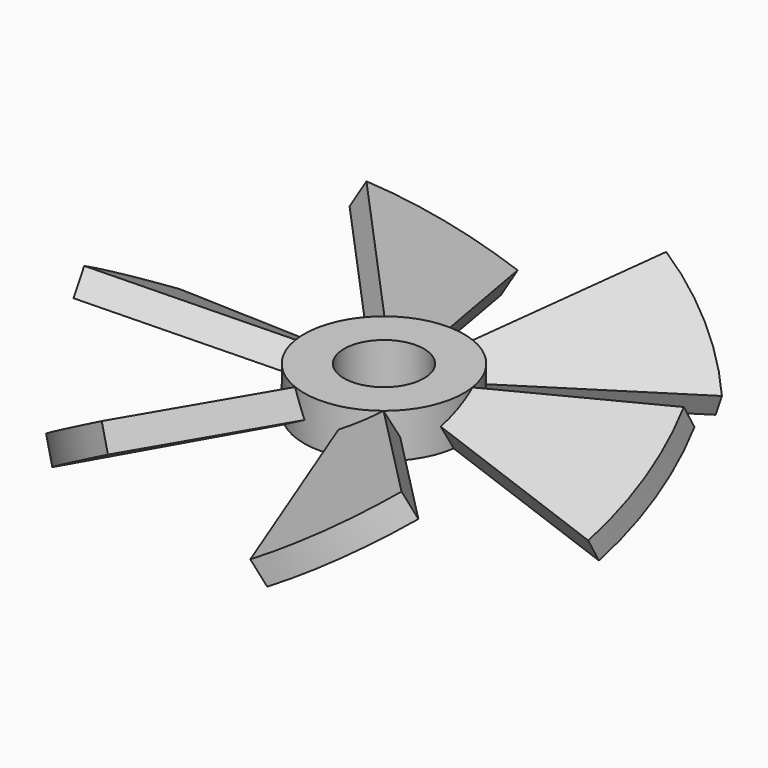
from build123d import *

# Parameters (mm, degrees)
F1_DEPTH  = 5
F2_ANGLE  = 30
F4_COUNT  = 6
F5_R      = 30
F6_DEPTH  = 12.5
F11_DEPTH = 4.1938354
F12_R     = 15
F13_DEPTH = 12.5


# Not quite as in the source:
# - an extrude ends at something that could not be found from the text; its depth is read off the source's solid
# - a feature of the source that left no trace in its solid (it failed there, or was rolled back) is left out
# - a pattern or mirror of a feature is missing from the dataset's text; its kind, count and spacing are read off the source's solid


with BuildPart() as f1:
    # F0 (on Top) → F1 (new body, symmetric)
    with BuildSketch(Plane.XY):
        with BuildLine():
            Line((96.5925826289, 25.8819045103), (0, 0))
            Line((0, 0), (96.5925826289, -25.8819045103))
            ThreePointArc((96.5925826289, -25.8819045103), (100, 0), (96.5925826289, 25.8819045103))
        make_face()
    extrude(amount=F1_DEPTH, both=True)


with BuildPart() as f1_1:
    # F2: moved
    add(f1.part.rotate(Axis((70.1462253928, 0, 0), (1, 0, 0)), F2_ANGLE))


with BuildPart() as f4_1:
    # F4: instance of F1
    add(f1_1.part.rotate(Axis((0, 0, 33.6874611676), (0, 0, 1)), 1 * 360 / F4_COUNT))


with BuildPart() as f4_2:
    # F4: instance of F1
    add(f1_1.part.rotate(Axis((0, 0, 33.6874611676), (0, 0, 1)), 2 * 360 / F4_COUNT))


with BuildPart() as f4_3:
    # F4: instance of F1
    add(f1_1.part.rotate(Axis((0, 0, 33.6874611676), (0, 0, 1)), 3 * 360 / F4_COUNT))


with BuildPart() as f4_4:
    # F4: instance of F1
    add(f1_1.part.rotate(Axis((0, 0, 33.6874611676), (0, 0, 1)), 4 * 360 / F4_COUNT))


with BuildPart() as f4_5:
    # F4: instance of F1
    add(f1_1.part.rotate(Axis((0, 0, 33.6874611676), (0, 0, 1)), 5 * 360 / F4_COUNT))


with BuildPart() as f1_2:
    add(f1_1.part)

    add(f4_1.part)  # F6 merges F4_1

    add(f4_2.part)  # F6 merges F4_2

    add(f4_3.part)  # F6 merges F4_3

    add(f4_4.part)  # F6 merges F4_4

    add(f4_5.part)  # F6 merges F4_5
    # F5 (on Top) → F6 (join, symmetric)
    with BuildSketch(Plane.XY):
        Circle(F5_R)
    extrude(amount=F6_DEPTH, both=True)

    # F11 (cut, through all): a face of the model
    f11_faces = [f1_2.faces().sort_by_distance(p)[0] for p in [
        (0, 0, -12.5),
    ]]
    f11 = extrude(f11_faces, amount=-F11_DEPTH, mode=Mode.SUBTRACT)

    # F11_copies: F11 across plane
    add(f11.mirror(Plane.XY), mode=Mode.SUBTRACT)

    # F12 (on Top) → F13 (cut, symmetric)
    with BuildSketch(Plane.XY):
        Circle(F12_R)
    extrude(amount=F13_DEPTH, both=True, mode=Mode.SUBTRACT)


solid = f1_2.part
